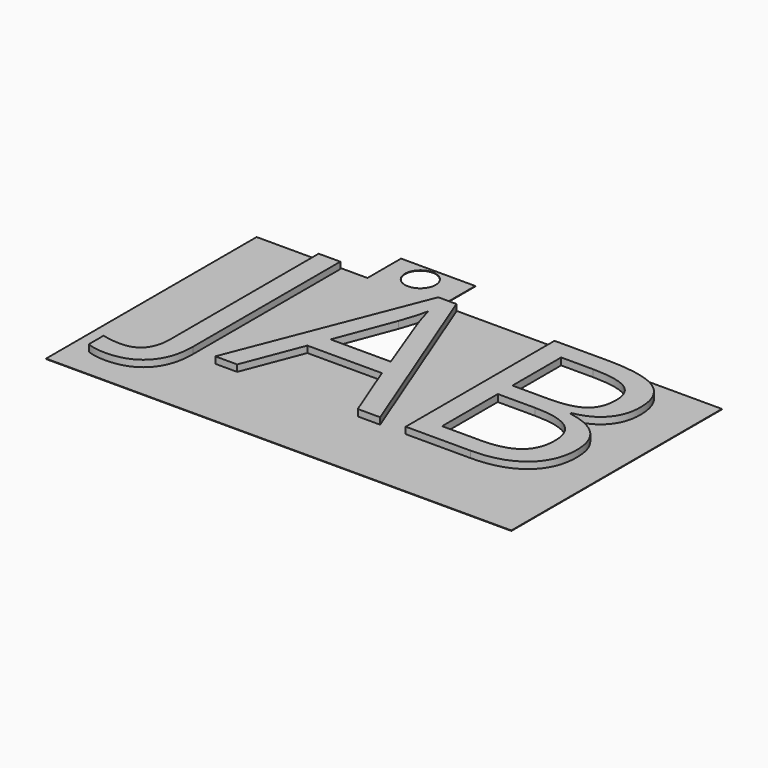
from build123d import *

# Parameters (mm, degrees)
F0_TEXT_SIZE = 140.8104267385
F1_DEPTH     = 3.81
F0_W         = 40.1022620499
F0_H         = 22.7169021964
F0_R         = 8.2713281546
F2_DEPTH     = 0.254


# Not quite as in the source:
# - Text() gives the source's letters only with a copy of the font that has no kerning and outlines rounded to 1/6400 em; it was checked with that copy


with BuildPart() as f1:
    # F0 (on Top) → F1 (new body)
    with BuildSketch(Plane.XY):
        with Locations((-54.0108531713, -45.8639711142)):
            Text('JAB', F0_TEXT_SIZE, font='Open Sans', text_align=(TextAlign.LEFT, TextAlign.BOTTOM))
    extrude(amount=F1_DEPTH)


with BuildPart() as f2:
    # F0 (on Top) → F2 (new body)
    with BuildSketch(Plane.XY):
        Polygon((-15.2717232704, 55.5195361376), (-54.0108531713, 55.5195361376), (-75.1655846834, 55.5195361376), (-75.1655846834, -86.7154300213), (176.3022010629, -86.7154300213), (176.3022010629, 55.5195361376), (24.8305387795, 55.5195361376), align=None)
        with BuildLine():
            add(Edge.make_bspline(
                [(-35.8595090996, -65.1483990886), (-42.459997853, -72.3319310152), (-54.8469150801, -72.3319310152)],
                knots=[0, 0, 0, 1, 1, 1], degree=2))
            add(Edge.make_bspline(
                [(-54.8469150801, -72.3319310152), (-61.2933924292, -72.3319310152), (-65.0116677603, -70.4837941642)],
                knots=[0, 0, 0, 1, 1, 1], degree=2))
            Line((-65.0116677603, -70.4837941642), (-65.0116677603, -60.5170561466))
            add(Edge.make_bspline(
                [(-65.0116677603, -60.5170561466), (-60.1273060828, -61.8811571557), (-54.8469150801, -61.8811571557)],
                knots=[0, 0, 0, 1, 1, 1], degree=2))
            add(Edge.make_bspline(
                [(-54.8469150801, -61.8811571557), (-48.026410035, -61.8811571557), (-44.4841477373, -57.7558516848)],
                knots=[0, 0, 0, 1, 1, 1], degree=2))
            add(Edge.make_bspline(
                [(-44.4841477373, -57.7558516848), (-40.9418854397, -53.630546214), (-40.9418854397, -45.8639711142)],
                knots=[0, 0, 0, 1, 1, 1], degree=2))
            Line((-40.9418854397, -45.8639711142), (-40.9418854397, 54.6614725996))
            Line((-40.9418854397, 54.6614725996), (-29.2590203462, 54.6614725996))
            Line((-29.2590203462, 54.6614725996), (-29.2590203462, -44.8958994303))
            add(Edge.make_bspline(
                [(-29.2590203462, -44.8958994303), (-29.2590203462, -57.964867162), (-35.8595090996, -65.1483990886)],
                knots=[0, 0, 0, 1, 1, 1], degree=2))
        make_face(mode=Mode.SUBTRACT)
        Polygon((72.6965292641, -45.8639711142), (60.5956332163, -45.8639711142), (48.0767062141, -13.8956039187), (7.7917231894, -13.8956039187), (-4.5731924086, -45.8639711142), (-16.4100689063, -45.8639711142), (23.324873389, 55.079503554), (33.1596016315, 55.079503554), align=None, mode=Mode.SUBTRACT)
        with BuildLine():
            Line((86.5135523879, -45.8639711142), (86.5135523879, 54.6614725996))
            Line((86.5135523879, 54.6614725996), (114.9176556565, 54.6614725996))
            add(Edge.make_bspline(
                [(114.9176556565, 54.6614725996), (134.9171365792, 54.6614725996), (143.86079884, 48.6770294633)],
                knots=[0, 0, 0, 1, 1, 1], degree=2))
            add(Edge.make_bspline(
                [(143.86079884, 48.6770294633), (152.8044611009, 42.6925863269), (152.8044611009, 29.7776299994)],
                knots=[0, 0, 0, 1, 1, 1], degree=2))
            add(Edge.make_bspline(
                [(152.8044611009, 29.7776299994), (152.8044611009, 20.822966924), (147.8210920921, 15.0145368211)],
                knots=[0, 0, 0, 1, 1, 1], degree=2))
            add(Edge.make_bspline(
                [(147.8210920921, 15.0145368211), (142.8377230833, 9.2061067181), (133.2670143909, 7.4899796422)],
                knots=[0, 0, 0, 1, 1, 1], degree=2))
            Line((133.2670143909, 7.4899796422), (133.2670143909, 6.8079291377))
            add(Edge.make_bspline(
                [(133.2670143909, 6.8079291377), (156.1707103651, 2.8916391441), (156.1707103651, -17.2618531829)],
                knots=[0, 0, 0, 1, 1, 1], degree=2))
            add(Edge.make_bspline(
                [(156.1707103651, -17.2618531829), (156.1707103651, -30.7268502398), (147.0620358854, -38.295410677)],
                knots=[0, 0, 0, 1, 1, 1], degree=2))
            add(Edge.make_bspline(
                [(147.0620358854, -38.295410677), (137.9533614058, -45.8639711142), (121.5841492974, -45.8639711142)],
                knots=[0, 0, 0, 1, 1, 1], degree=2))
            Line((121.5841492974, -45.8639711142), (86.5135523879, -45.8639711142))
        make_face(mode=Mode.SUBTRACT)
        with Locations((4.7794077545, 66.8779872358)):
            Rectangle(F0_W, F0_H)
        with Locations((2.8996153269, 68.5241743922)):
            Circle(F0_R, mode=Mode.SUBTRACT)
    extrude(amount=F2_DEPTH)


solid = Compound([f1.part, f2.part])
